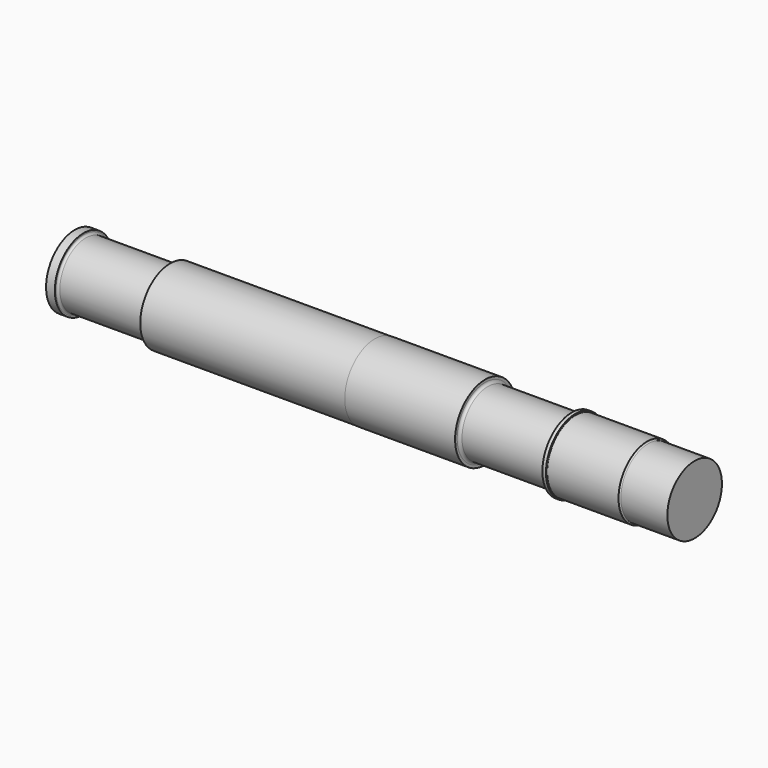
from build123d import *


# Not quite as in the source:
# - a feature names something its author has since deleted; it is built from what else it names


with BuildPart() as f1:
    # F0 (on Front) → F1 (revolve)
    with BuildSketch(Plane.XZ):
        Polygon((259, 254), (259, 0), (321, 0), (321, 243.6), (321, 254), align=None)
        Polygon((933.8, 243.6), (933.8, 0), (2380.8, 0), (2380.8, 261), (2380.8, 265), (933.8, 265), align=None)
        Polygon((2380.8, 261), (2380.8, 0), (3160.8, 0), (3160.8, 247.6), (3160.8, 266), (2380.8, 266), (2380.8, 265), align=None)
        with BuildLine():
            Line((3160.8, 247.6), (3160.8, 0))
            Line((3160.8, 0), (3773.6, 0))
            Line((3773.6, 0), (3773.6, 247.6))
            ThreePointArc((3773.6, 247.6), (3768.0350288425, 234.1649711575), (3754.6, 228.6))
            Line((3754.6, 228.6), (3179.8, 228.6))
            ThreePointArc((3179.8, 228.6), (3166.3649711575, 234.1649711575), (3160.8, 247.6))
        make_face()
        with BuildLine():
            Line((3799, 255.2237437367), (3799, 0))
            Line((3799, 0), (4305.4, 0))
            Line((4305.4, 0), (4305.4, 249.3))
            Line((4305.4, 249.3), (4305.4, 252.2237437367))
            Line((4305.4, 252.2237437367), (3802, 252.2237437367))
            ThreePointArc((3802, 252.2237437367), (3799.8786796564, 253.1024233932), (3799, 255.2237437367))
        make_face()
        Polygon((3773.6, 247.6), (3773.6, 0), (3799, 0), (3799, 255.2237437367), (3799, 260.35), (3773.6, 260.35), align=None)
        with BuildLine():
            Line((4305.4, 249.3), (4305.4, 0))
            Line((4305.4, 0), (4641.95, 0))
            Line((4641.95, 0), (4641.95, 241.3))
            Line((4641.95, 241.3), (4313.4, 241.3))
            ThreePointArc((4313.4, 241.3), (4307.7431457505, 243.6431457505), (4305.4, 249.3))
        make_face()
        with BuildLine():
            Line((321, 243.6), (321, 0))
            Line((321, 0), (933.8, 0))
            Line((933.8, 0), (933.8, 243.6))
            ThreePointArc((933.8, 243.6), (929.4066017178, 232.9933982822), (918.8, 228.6))
            Line((918.8, 228.6), (336, 228.6))
            ThreePointArc((336, 228.6), (325.3933982822, 232.9933982822), (321, 243.6))
        make_face()
    revolve(axis=Axis((23207.5, 0, 0), (1, 0, 0)))


with BuildPart() as f1_1:
    # F2: moved
    add(f1.part.moved(Location((0, 0, 862.5))))


solid = f1_1.part
